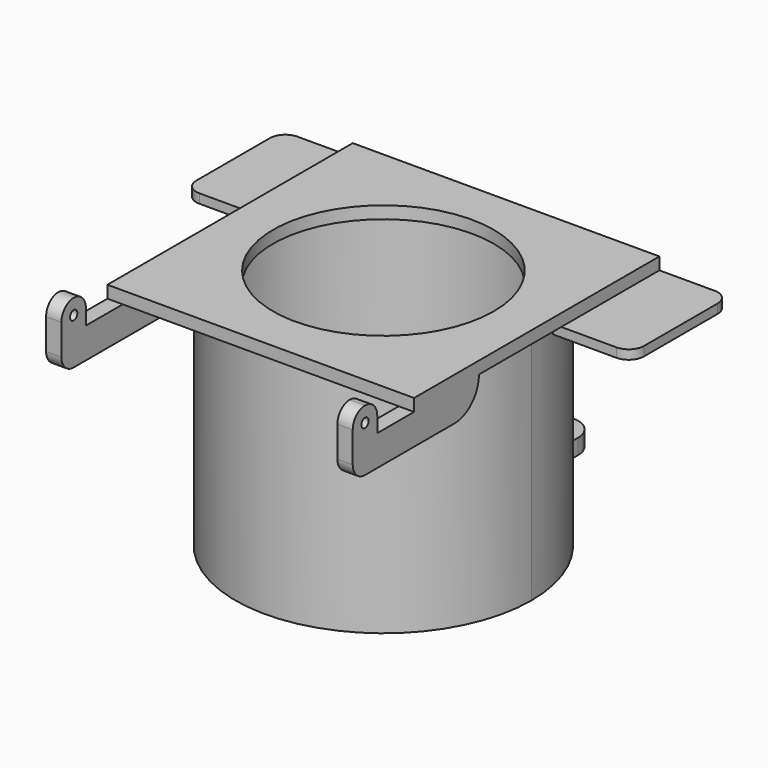
from build123d import *

# Parameters (mm, degrees)
F0_R      = 45.3
F1_DEPTH  = 75
F2_DEPTH  = 5
F3_R      = 2.5
F4_DEPTH  = 3
F5_W      = 100
F5_H      = 100
F5_R      = 48.3
F5_R_2    = 45.3
F5_R_3    = 36
F6_DEPTH  = 4
F8_DEPTH  = 3
F9_W      = 5
F9_H      = 26.435303688
F9_H_2    = 20
F10_DEPTH = 10
F12_DEPTH = 5
F14_DEPTH = 5
F15_R     = 5
F16_R     = 4.99999
F17_R     = 1.5
F18_DEPTH = 5
F20_R     = 1.5
F21_DEPTH = 5


# Not quite as in the source:
# - a fillet or chamfer is up to 0.001 mm smaller than in the source, because OpenCascade refuses the exact size


with BuildPart() as f1:
    # F0 (on Top) → F1 (new body)
    with BuildSketch(Plane.XY):
        with BuildLine():
            ThreePointArc((-7.5, 47.714148845), (-31.3898072629, -36.7092631362), (48.3, 0))
            ThreePointArc((48.3, 0), (36.7092631362, 31.3898072629), (7.5, 47.714148845))
            Line((7.5, 47.714148845), (7.5, 46.6673743725))
            Line((7.5, 46.6673743725), (-7.5, 46.6673743725))
            Line((-7.5, 46.6673743725), (-7.5, 47.714148845))
        make_face()
        Circle(F0_R, mode=Mode.SUBTRACT)
        with BuildLine():
            Line((7.5, 46.6673743725), (7.5, 47.714148845))
            ThreePointArc((7.5, 47.714148845), (0, 48.3), (-7.5, 47.714148845))
            Line((-7.5, 47.714148845), (-7.5, 46.6673743725))
            Line((-7.5, 46.6673743725), (7.5, 46.6673743725))
        make_face()
    extrude(amount=F1_DEPTH)

    # F0 (on Top) → F2 (join)
    with BuildSketch(Plane.XY):
        with BuildLine():
            ThreePointArc((-7.5, 47.714148845), (-31.3898072629, -36.7092631362), (48.3, 0))
            ThreePointArc((48.3, 0), (36.7092631362, 31.3898072629), (7.5, 47.714148845))
            Line((7.5, 47.714148845), (7.5, 46.6673743725))
            Line((7.5, 46.6673743725), (-7.5, 46.6673743725))
            Line((-7.5, 46.6673743725), (-7.5, 47.714148845))
        make_face()
        Circle(F0_R, mode=Mode.SUBTRACT)
        with BuildLine():
            Line((7.5, 46.6673743725), (7.5, 47.714148845))
            ThreePointArc((7.5, 47.714148845), (0, 48.3), (-7.5, 47.714148845))
            Line((-7.5, 47.714148845), (-7.5, 46.6673743725))
            Line((-7.5, 46.6673743725), (7.5, 46.6673743725))
        make_face()
        with BuildLine():
            ThreePointArc((-7.5, 47.714148845), (0, 48.3), (7.5, 47.714148845))
            Line((7.5, 47.714148845), (7.5, 70))
            ThreePointArc((7.5, 70), (0, 77.5), (-7.5, 70))
            Line((-7.5, 70), (-7.5, 47.714148845))
        make_face()
    extrude(amount=F2_DEPTH)

    # F3 (on face) → F4 (cut)
    with BuildSketch(Plane.XY.offset(5)):
        with Locations((0, 70)):
            Circle(F3_R)
    extrude(amount=-F4_DEPTH, mode=Mode.SUBTRACT)

    # F5 (on face) → F6 (join)
    with BuildSketch(Plane.XY.offset(75)):
        Rectangle(F5_W, F5_H)
        Circle(F5_R, mode=Mode.SUBTRACT)
        Circle(F5_R)
        Circle(F5_R_2, mode=Mode.SUBTRACT)
        Circle(F5_R_2)
        Circle(F5_R_3, mode=Mode.SUBTRACT)
    extrude(amount=F6_DEPTH)

    # F7 (on face) → F8 (join)
    with BuildSketch(Plane(origin=(0, 0, 75), x_dir=(1, 0, 0), z_dir=(0, 0, -1))):
        with BuildLine():
            Line((-68, -50), (-45.938372612, -50))
            Line((-45.938372612, -50), (-34.8247885738, -50))
            ThreePointArc((-34.8247885738, -50), (-30.5975043414, -47.6702187211), (-30.3096791752, -42.8520272073))
            Line((-30.3096791752, -42.8520272073), (-45.938372612, -10))
            Line((-45.938372612, -10), (-68, -10))
            ThreePointArc((-68, -10), (-71.5355339059, -11.4644660941), (-73, -15))
            Line((-73, -15), (-73, -45))
            ThreePointArc((-73, -45), (-71.5355339059, -48.5355339059), (-68, -50))
        make_face()
        with BuildLine():
            Line((68, -10), (45.938372612, -10))
            Line((45.938372612, -10), (30.3096791752, -42.8520272073))
            ThreePointArc((30.3096791752, -42.8520272073), (30.5975043414, -47.6702187211), (34.8247885738, -50))
            Line((34.8247885738, -50), (45.938372612, -50))
            Line((45.938372612, -50), (68, -50))
            ThreePointArc((68, -50), (71.5355339059, -48.5355339059), (73, -45))
            Line((73, -45), (73, -15))
            ThreePointArc((73, -15), (71.5355339059, -11.4644660941), (68, -10))
        make_face()
    extrude(amount=F8_DEPTH)

    # F9 (on face) → F10 (join)
    with BuildSketch(Plane(origin=(0, 0, 75), x_dir=(1, 0, 0), z_dir=(0, 0, -1))):
        with Locations((47.5, 36.782348156)):
            Rectangle(F9_W, F9_H)
        with Locations((47.5, 60)):
            Rectangle(F9_W, F9_H_2)
    extrude(amount=F10_DEPTH)

    # F11 (on face) → F12 (cut, through all)
    with BuildSketch(Plane.YZ.offset(50)):
        with BuildLine():
            ThreePointArc((-23.564696312, 75), (-26.3246425928, 68.0971789948), (-33.0828763545, 65))
            Line((-33.0828763545, 65), (-23.564696312, 65))
            Line((-23.564696312, 65), (-23.564696312, 75))
        make_face()
    extrude(amount=-F12_DEPTH, mode=Mode.SUBTRACT)

    # F13 (on face) → F14 (join)
    with BuildSketch(Plane.YZ.offset(50)):
        Polygon((-70, 65), (-70, 75), (-65, 75), (-65, 85), (-75, 85), (-75, 65), align=None)
    extrude(amount=-F14_DEPTH)

    # F15
    f15_edges = [f1.edges().sort_by_distance(p)[0] for p in [
        (47.5, -75, 65),
    ]]
    fillet(f15_edges, radius=F15_R)

    # F16 (radius 5 in the source; OpenCascade refuses exactly that, so slightly less here)
    f16_edges = [f1.edges().sort_by_distance(p)[0] for p in [
        (47.5, -75, 85),
        (47.5, -65, 85),
    ]]
    fillet(f16_edges, radius=F16_R)

    # F17 (on face) → F18 (cut, through all)
    with BuildSketch(Plane.YZ.offset(50)):
        with Locations((-70, 80)):
            Circle(F17_R)
    extrude(amount=-F18_DEPTH, mode=Mode.SUBTRACT)

    # F20 (on offset) → F21 (join)
    with BuildSketch(Plane(origin=(-50, 0, 0), x_dir=(0, -1, 0), z_dir=(-1, 0, 0))):
        with BuildLine():
            Line((75, 70), (75, 80))
            ThreePointArc((75, 80), (70, 85), (65, 80))
            Line((65, 80), (65, 75))
            Line((65, 75), (50, 75))
            Line((50, 75), (23.564696312, 75))
            ThreePointArc((23.564696312, 75), (26.3246425928, 68.0971789948), (33.0828763545, 65))
            Line((33.0828763545, 65), (70, 65))
            ThreePointArc((70, 65), (73.5355339059, 66.4644660941), (75, 70))
        make_face()
        with Locations((70, 80)):
            Circle(F20_R, mode=Mode.SUBTRACT)
    extrude(amount=-F21_DEPTH)


solid = f1.part
